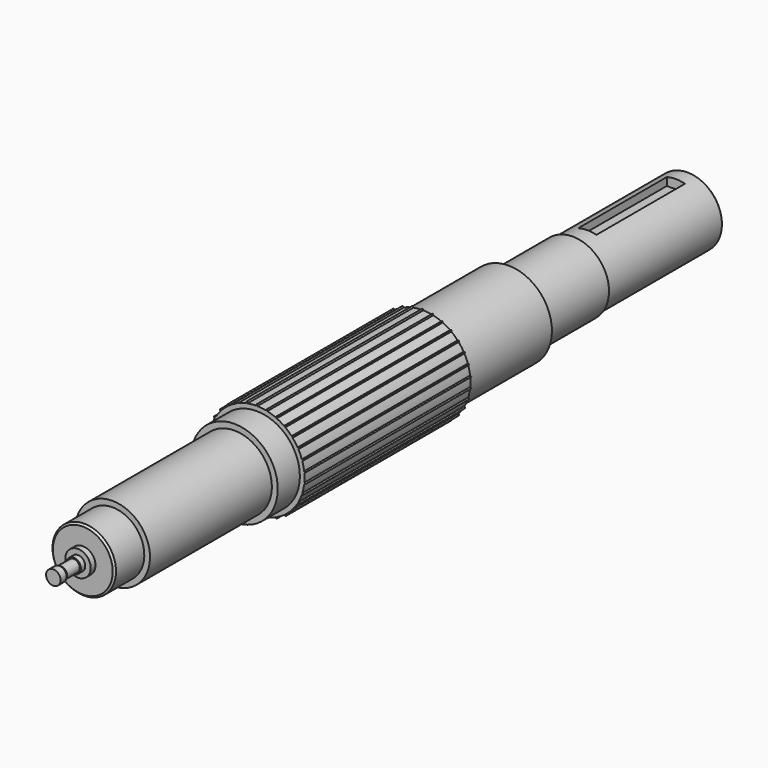
from build123d import *

# Parameters (mm, degrees)
F3_DEPTH        = 254.2296
F3_COPIES_COUNT = 30
F6_DEPTH        = 5
F7_SIZE         = 1.016


# Not quite as in the source:
# - a pattern or mirror of a feature is missing from the dataset's text; its kind, count and spacing are read off the source's solid


with BuildPart() as f1:
    # F0 (on Right) → F1 (revolve)
    with BuildSketch(Plane.YZ):
        Polygon((59.2582, 23.876), (0, 23.876), (0, 27.1526), (-114.3, 27.1526), (-114.3, 23.876), (-129.54, 23.876), (-129.54, 20.6375), (-213.4616, 20.6375), (-213.4616, 17.5006), (-233.934, 17.5006), (-233.934, 6.985), (-237.236, 6.985), (-237.236, 3.99415), (-240.2332, 3.99415), (-240.2332, 3.3655), (-248.9962, 3.3655), (-250.0850537402, 3.99415), (-254.2286, 3.99415), (-254.2286, 0), (-233.934, 0), (183.4388, 0), (183.4388, 18.9992), (103.4288, 18.9992), (103.4288, 19.9898), (59.2582, 19.9898), align=None)
    revolve(axis=Axis((0, -25.2476, 0), (0, 1, 0)))

    # F2 (on face) → F3 (cut, through all)
    with BuildSketch(Plane(origin=(0, 0, 0), x_dir=(-1, 0, 0), z_dir=(0, 1, 0))):
        with BuildLine():
            Line((-0.442078818, 26.3868970263), (0, 27.1526))
            ThreePointArc((0, 27.1526), (-2.8382195517, 27.0038552162), (-5.6453429761, 26.5592505437))
            Line((-5.6453429761, 26.5592505437), (-5.0537260411, 25.9021933716))
            ThreePointArc((-5.0537260411, 25.9021933716), (-2.7585688627, 26.2460295319), (-0.442078818, 26.3868970263))
        make_face()
    f3 = extrude(amount=-F3_DEPTH, mode=Mode.SUBTRACT)

    # F3_copies: F3 ×30 about axis
    f3_copies_axis = Axis((0, 0, 0), (0, 1, 0))
    for i in range(1, F3_COPIES_COUNT):
        add(f3.rotate(f3_copies_axis, i * 360 / F3_COPIES_COUNT), mode=Mode.SUBTRACT)

    # F5 (on offset) → F6 (cut)
    with BuildSketch(Plane.XY.offset(18.9992)):
        Polygon((-4.99999, 174.4472), (-4.99999, 113.4872), (4.99999, 113.4872), (4.99999, 174.4472), (0, 174.4472), align=None)
    extrude(amount=-F6_DEPTH, mode=Mode.SUBTRACT)

    # F7
    f7_edges = [f1.edges().sort_by_distance(p)[0] for p in [
        (0, 183.4388, -18.9992),
        (0, -233.934, -17.5006),
    ]]
    chamfer(f7_edges, length=F7_SIZE)


solid = f1.part
